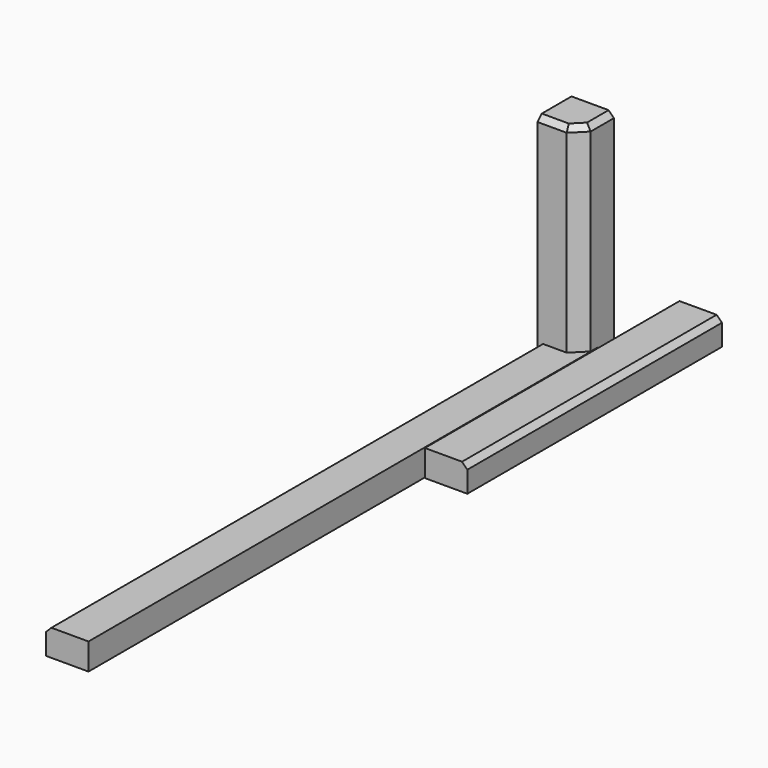
from build123d import *

# Parameters (mm, degrees)
F0_W     = 80
F0_H     = 80
F1_DEPTH = 400
F2_SIZE  = 25
F3_SIZE  = 10
F4_W     = 80
F4_H     = 50
F5_DEPTH = 600
F6_W     = 80
F6_H     = 50
F7_DEPTH = 1200
F8_SIZE  = 10
F9_SIZE  = 10


with BuildPart() as f1:
    # F0 (on Top) → F1 (new body)
    with BuildSketch(Plane.XY):
        with Locations((-0.3851265647, -1.187727477)):
            Rectangle(F0_W, F0_H)
    extrude(amount=F1_DEPTH)

    # F2
    f2_edges = [f1.edges().sort_by_distance(p)[0] for p in [
        (39.614873, -41.187727, 200),
    ]]
    chamfer(f2_edges, length=F2_SIZE)

    # F3
    f3_edges = [f1.edges().sort_by_distance(p)[0] for p in [
        (-12.885127, -41.187727, 400),
        (39.614873, 11.312273, 400),
        (27.114873, -28.687727, 400),
    ]]
    chamfer(f3_edges, length=F3_SIZE)


with BuildPart() as f5:
    # F4 (on Front) → F5 (new body)
    with BuildSketch(Plane.XZ):
        with Locations((234.2652007937, 127.4122001697)):
            Rectangle(F4_W, F4_H)
    extrude(amount=F5_DEPTH)

    # F8
    f8_edges = [f5.edges().sort_by_distance(p)[0] for p in [
        (274.265201, -300, 152.4122),
    ]]
    chamfer(f8_edges, length=F8_SIZE)


with BuildPart() as f7:
    # F6 (on Front) → F7 (new body)
    with BuildSketch(Plane.XZ):
        Rectangle(F6_W, F6_H)
    extrude(amount=F7_DEPTH)

    # F9
    f9_edges = [f7.edges().sort_by_distance(p)[0] for p in [
        (-40, -600, 25),
    ]]
    chamfer(f9_edges, length=F9_SIZE)


solid = Compound([f1.part, f5.part, f7.part])
